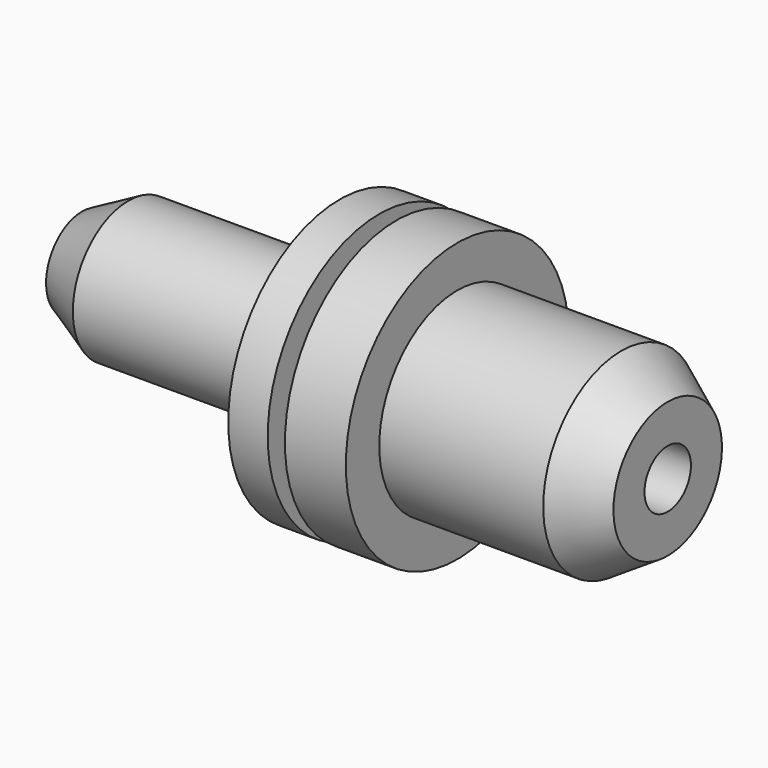
from build123d import *
from build123d import SkipClean  # not in build123d's __all__

# Parameters (mm, degrees)
F0_R     = 9.49325
F1_DEPTH = 35.2425
F2_R     = 19.05
F3_DEPTH = 16.0782
F4_R     = 13.335
F5_DEPTH = 28.7655
F6_R     = 3.96875
F7_DEPTH = 80.0862
F8_R     = 16.51
F8_R_2   = 9.49325
F9_DEPTH = 2.0955
F10_W    = 3.81
F10_H    = 0.508
F12_W    = 2.3495
F12_H    = 4.4069


with BuildPart() as f1:
    # F0 (on Right) → F1 (new body)
    with BuildSketch(Plane.YZ):
        Circle(F0_R)
    extrude(amount=F1_DEPTH)

    # F2 (on face) → F3 (join)
    with BuildSketch(Plane.YZ.offset(35.2425)):
        Circle(F2_R)
    extrude(amount=F3_DEPTH)

    # F4 (on face) → F5 (join)
    with BuildSketch(Plane.YZ.offset(51.3207)):
        Circle(F4_R)
    extrude(amount=F5_DEPTH)

    # F6 (on face) → F7 (cut, through all)
    with BuildSketch(Plane.YZ.offset(80.0862)):
        Circle(F6_R)
    extrude(amount=-F7_DEPTH, mode=Mode.SUBTRACT)

    # F8 (on face) → F9 (cut)
    with BuildSketch(Plane(origin=(35.2425, 0, 0), x_dir=(0, -1, 0), z_dir=(-1, 0, 0))):
        Circle(F8_R)
        Circle(F8_R_2, mode=Mode.SUBTRACT)
    with SkipClean():  # cleaning this boolean's faces spoils the solid; the shape is the same uncleaned
        extrude(amount=-F9_DEPTH, mode=Mode.SUBTRACT)

    # F10 (on Front) → F11 (revolve, cut)
    with BuildSketch(Plane.XZ):
        with Locations((36.0383225369, 9.23925)):
            Rectangle(F10_W, F10_H)
    revolve(axis=Axis((43.7559969723, 0, 0), (1, 0, 0)), mode=Mode.SUBTRACT)

    # F12 (on Front) → F13 (revolve, cut)
    with BuildSketch(Plane.XZ):
        with Locations((41.81475, 16.84655)):
            Rectangle(F12_W, F12_H)
    revolve(axis=Axis((42.9936237633, 0, 0), (1, 0, 0)), mode=Mode.SUBTRACT)

    # F14 (on Front) → F15 (revolve, cut)
    with BuildSketch(Plane.XZ):
        Polygon((6.35, 9.49325), (0, 9.49325), (0, 6.12775), align=None)
        Polygon((80.0862, 13.335), (73.7362, 13.335), (80.0862, 9.271), align=None)
    revolve(axis=Axis((41.732724756, 0, 0), (1, 0, 0)), mode=Mode.SUBTRACT)


solid = f1.part
